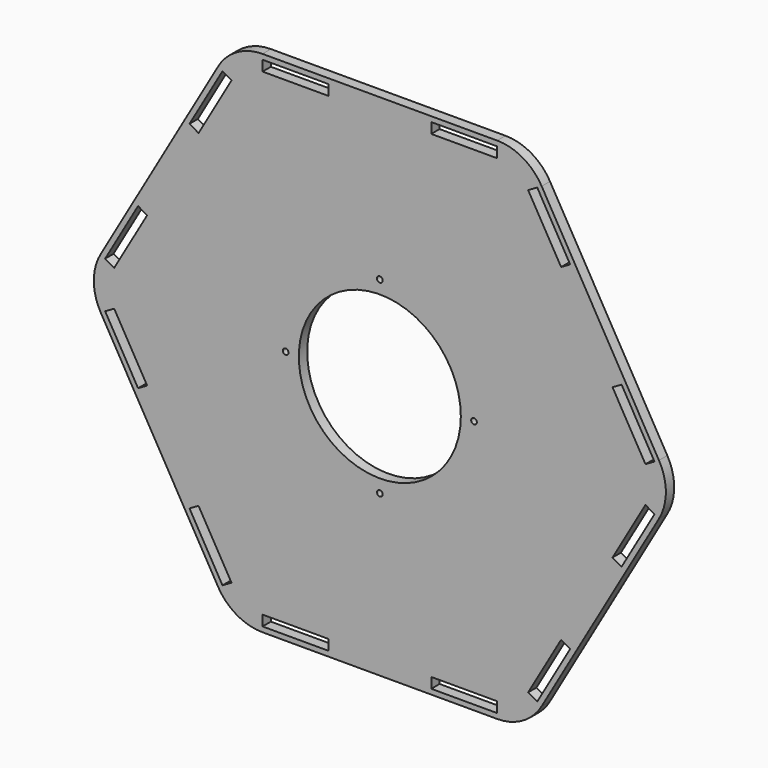
from build123d import *

# Parameters (mm, degrees)
F1_DEPTH        = 5.1562
F2_R            = 40.005
F2_R_2          = 1.397
F3_DEPTH        = 5.1572
F4_W            = 32.5247
F4_H            = 5.1562
F5_DEPTH        = 5.1572
F5_COPIES_COUNT = 6


# Not quite as in the source:
# - a pattern or mirror of a feature is missing from the dataset's text; its kind, count and spacing are read off the source's solid


with BuildPart() as f1:
    # F0 (on Front) → F1 (new body)
    with BuildSketch(Plane.XZ):
        with BuildLine():
            Line((137.8481502717, 12.7), (79.9225977639, 113.03))
            ThreePointArc((79.9225977639, 113.03), (70.6255525078, 122.3270452561), (57.9255525078, 125.73))
            Line((57.9255525078, 125.73), (-57.9255525078, 125.73))
            ThreePointArc((-57.9255525078, 125.73), (-70.6255525078, 122.3270452561), (-79.9225977639, 113.03))
            Line((-79.9225977639, 113.03), (-137.8481502717, 12.7))
            ThreePointArc((-137.8481502717, 12.7), (-141.2511050156, 0), (-137.8481502717, -12.7))
            Line((-137.8481502717, -12.7), (-79.9225977639, -113.03))
            ThreePointArc((-79.9225977639, -113.03), (-70.6255525078, -122.3270452561), (-57.9255525078, -125.73))
            Line((-57.9255525078, -125.73), (57.9255525078, -125.73))
            ThreePointArc((57.9255525078, -125.73), (70.6255525078, -122.3270452561), (79.9225977639, -113.03))
            Line((79.9225977639, -113.03), (137.8481502717, -12.7))
            ThreePointArc((137.8481502717, -12.7), (141.2511050156, 0), (137.8481502717, 12.7))
        make_face()
    extrude(amount=-F1_DEPTH)

    # F2 (on face) → F3 (cut, through all)
    with BuildSketch(Plane.XZ):
        Circle(F2_R)
        with Locations((0, 46.4947)):
            Circle(F2_R_2)
        with Locations((-46.4947, 0)):
            Circle(F2_R_2)
        with Locations((0, -46.4947)):
            Circle(F2_R_2)
        with Locations((46.4947, 0)):
            Circle(F2_R_2)
    extrude(amount=-F3_DEPTH, mode=Mode.SUBTRACT)

    # F4 (on face) → F5 (cut, through all)
    with BuildSketch(Plane.XZ):
        with Locations((-41.66235, 120.6119)):
            Rectangle(F4_W, F4_H)
        with Locations((41.66235, 120.6119)):
            Rectangle(F4_W, F4_H)
    f5 = extrude(amount=-F5_DEPTH, mode=Mode.SUBTRACT)

    # F5_copies: F5 ×6 about axis
    f5_copies_axis = Axis((0, 0, 0), (0, 1, 0))
    for i in range(1, F5_COPIES_COUNT):
        add(f5.rotate(f5_copies_axis, i * 360 / F5_COPIES_COUNT), mode=Mode.SUBTRACT)


solid = f1.part
